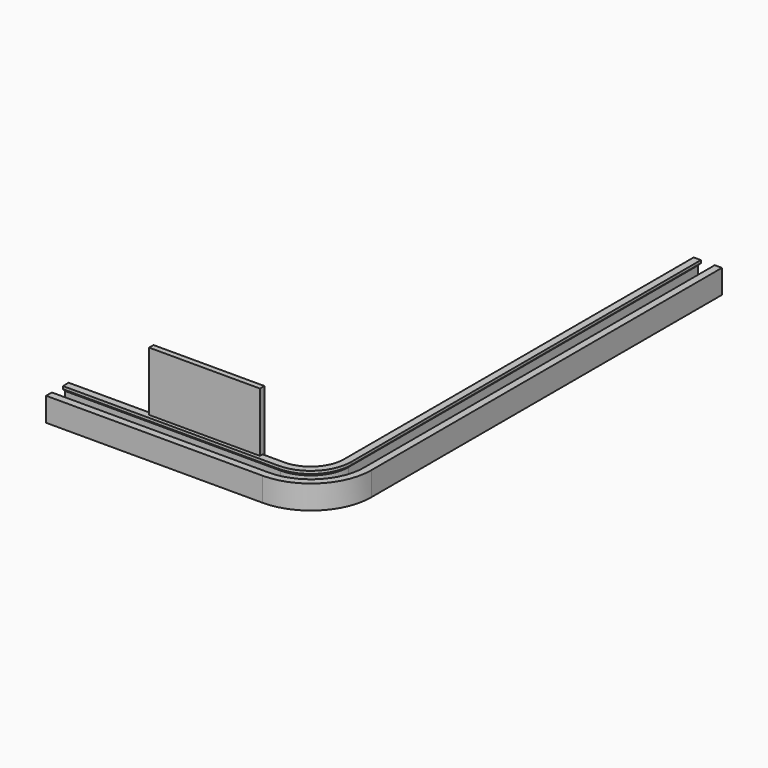
from build123d import *

# Parameters (mm, degrees)
F1_DEPTH = 8.6
F2_R     = 12
F3_R     = 21.8
F4_T     = -1.6
F6_DEPTH = 2
F7_SIZE  = 0.99999
F8_W     = 40
F8_H     = 2
F9_DEPTH = 30


# Not quite as in the source:
# - a fillet or chamfer is up to 0.001 mm smaller than in the source, because OpenCascade refuses the exact size


with BuildPart() as f1:
    # F0 (on Top) → F1 (new body)
    with BuildSketch(Plane.XY):
        Polygon((0, 0), (0, 180), (-10.2, 180), (-10.2, 10.2), (-100, 10.2), (-100, 0), align=None)
    extrude(amount=F1_DEPTH)

    # F2
    f2_edges = [f1.edges().sort_by_distance(p)[0] for p in [
        (-10.2, 10.2, 4.3),
    ]]
    fillet(f2_edges, radius=F2_R)

    # F3
    f3_edges = [f1.edges().sort_by_distance(p)[0] for p in [
        (0, 0, 4.3),
    ]]
    fillet(f3_edges, radius=F3_R)

    # F4
    f4_openings = [f1.faces().sort_by_distance(p)[0] for p in [
        (-100, 5.1, 4.3),
        (-2.059126, 100.9, 8.6),
        (-5.1, 180, 4.3),
    ]]
    offset(amount=F4_T, openings=f4_openings)

    # F5 (on face) → F6 (join)
    with BuildSketch(Plane.XY.offset(8.6)):
        with BuildLine():
            ThreePointArc((-22.2, 7.6), (-11.8762409947, 11.8762409947), (-7.6, 22.2))
            Line((-7.6, 22.2), (-7.6, 180))
            Line((-7.6, 180), (-10.2, 180))
            Line((-10.2, 180), (-10.2, 22.2))
            ThreePointArc((-10.2, 22.2), (-13.7147186258, 13.7147186258), (-22.2, 10.2))
            Line((-22.2, 10.2), (-100, 10.2))
            Line((-100, 10.2), (-100, 7.6))
            Line((-100, 7.6), (-22.2, 7.6))
        make_face()
        with BuildLine():
            Line((0, 21.8), (0, 180))
            Line((0, 180), (-2.6, 180))
            Line((-2.6, 180), (-2.6, 21.8))
            ThreePointArc((-2.6, 21.8), (-8.2235498012, 8.2235498012), (-21.8, 2.6))
            Line((-21.8, 2.6), (-100, 2.6))
            Line((-100, 2.6), (-100, 0))
            Line((-100, 0), (-21.8, 0))
            ThreePointArc((-21.8, 0), (-6.3850721701, 6.3850721701), (0, 21.8))
        make_face()
    extrude(amount=-F6_DEPTH)

    # F7 (size 1 in the source; OpenCascade refuses exactly that, so slightly less here)
    f7_edges = [f1.edges().sort_by_distance(p)[0] for p in [
        (-61.1, 7.6, 6.6),
        (-60.9, 2.6, 6.6),
    ]]
    chamfer(f7_edges, length=F7_SIZE)

    # F8 (on Top) → F9 (join)
    with BuildSketch(Plane.XY):
        with Locations((-50, 10)):
            Rectangle(F8_W, F8_H)
    extrude(amount=F9_DEPTH)


solid = f1.part
